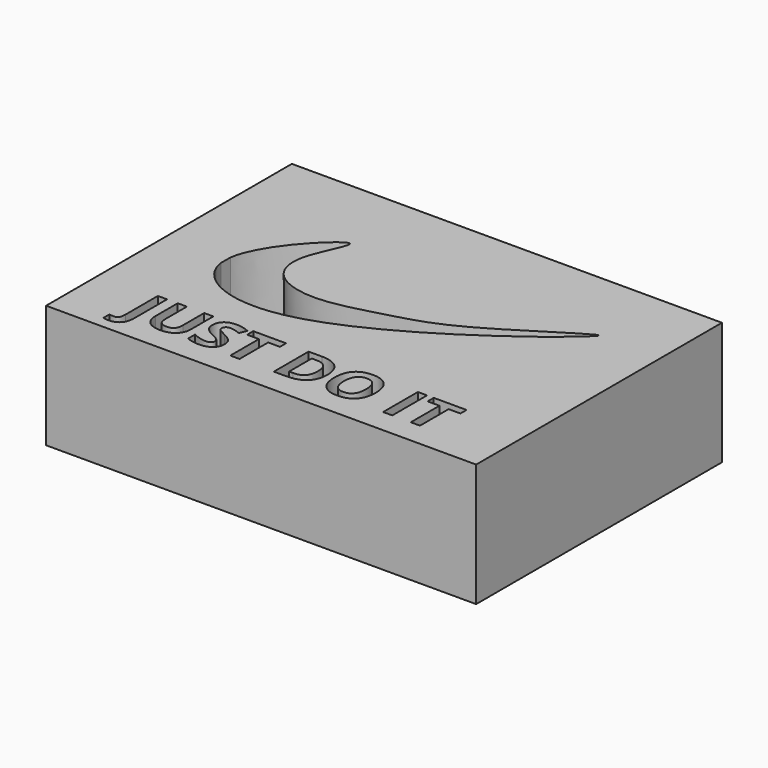
from build123d import *

# Parameters (mm, degrees)
F1_W         = 50
F1_H         = 25
F2_DEPTH     = 20
F0_W         = 70
F0_H         = 50
F4_DEPTH     = 20
F5_DEPTH     = 10
F6_TEXT_SIZE = 9.9044344905
F7_DEPTH     = 10


# Not quite as in the source:
# - Text() gives the source's letters only with a copy of the font that has no kerning and outlines rounded to 1/6400 em; it was checked with that copy


with BuildPart() as f2:
    # F1 (on face) → F2 (new body)
    with BuildSketch(Plane.XY):
        Rectangle(F1_W, F1_H)
    extrude(amount=F2_DEPTH)

    # F0 (on Top) → F4 (join)
    with BuildSketch(Plane.XY):
        Rectangle(F0_W, F0_H)
    extrude(amount=F4_DEPTH)

    # F3 (on face) → F5 (cut)
    with BuildSketch(Plane.XY.offset(20)):
        with BuildLine():
            add(Edge.make_bspline(
                [(24.768707636, 12.5), (23.3617196124, 11.9913440467), (8.9697295179, 2.129022155), (0.6864078964, 0.3295618388), (-9.0991916536, -2.7306011387), (-16.9481476968, -0.8251153414), (-19.1678494539, 5.3334645726), (-14.8813581254, 12.2781949204), (-15.5801502988, 12.5)],
                knots=[0.4528338424, 0.4528338424, 0.4528338424, 0.4528338424, 0.5654700584, 0.6685449092, 0.7628214115, 0.8442260701, 0.9193712141, 1, 1, 1, 1], degree=3))
            Line((-15.5801502988, 12.5), (-15.7586222597, 12.5))
            add(Edge.make_bspline(
                [(-15.7586222597, 12.5), (-17.2907082648, 12.1887744552), (-24.2406929756, 5.3595854924), (-25, 0)],
                knots=[0.0054001273, 0.0054001273, 0.0054001273, 0.0054001273, 0.120658891, 0.120658891, 0.120658891, 0.120658891], degree=3))
            Line((-25, 0), (-25, -1.9452686889))
            add(Edge.make_bspline(
                [(-25, -1.9452686889), (-24.2830336658, -6.728801974), (-7.60312682, -15.0152890661), (24.9264006489, 11.4585565306), (25, 12.489551636)],
                knots=[0.1351481492, 0.1351481492, 0.1351481492, 0.1351481492, 0.2467620308, 0.4404103146, 0.4404103146, 0.4404103146, 0.4404103146], degree=3))
            Line((25, 12.489551636), (25, 12.5))
            Line((25, 12.5), (24.768707636, 12.5))
        make_face()
    extrude(amount=-F5_DEPTH, mode=Mode.SUBTRACT)

    # F6 (on face) → F7 (cut)
    with BuildSketch(Plane.XY.offset(20)):
        with Locations((-26.4809280634, -21.0950635374)):
            Text('JUST DO IT', F6_TEXT_SIZE, font='Open Sans', font_style=FontStyle.BOLD, text_align=(TextAlign.LEFT, TextAlign.BOTTOM))
    extrude(amount=-F7_DEPTH, mode=Mode.SUBTRACT)


solid = f2.part
